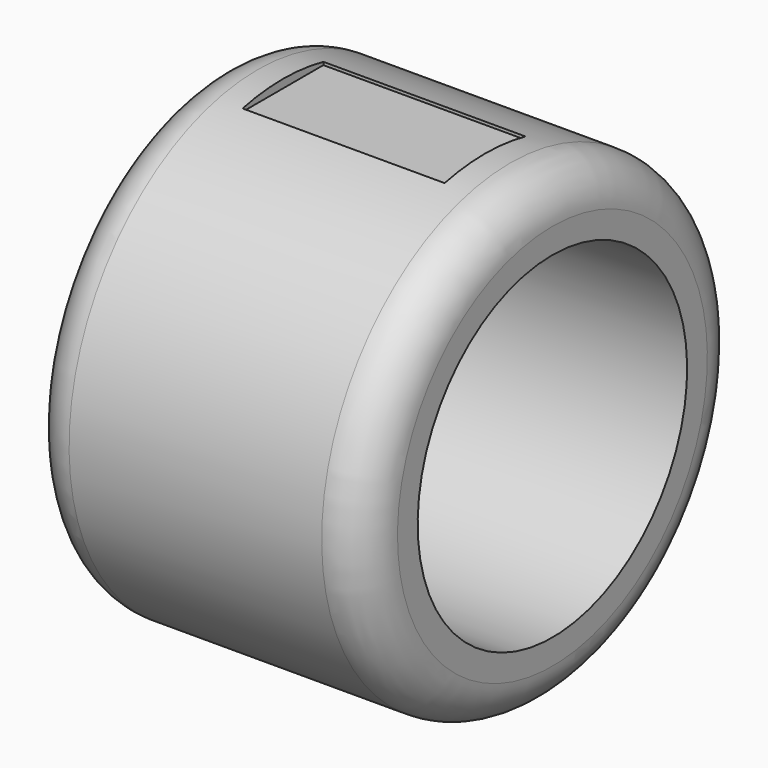
from build123d import *

# Parameters (mm, degrees)
F0_W     = 24
F0_H     = 1
F2_R     = 5
F3_DEPTH = 6


with BuildPart() as f1:
    # F0 (on Front) → F1 (revolve)
    with BuildSketch(Plane.XZ):
        Polygon((-20, 28), (-20, 20), (0, 20), (20, 20), (20, 28), (12, 28), (12, 27), (-12, 27), (-12, 28), align=None)
        with Locations((0, 27.5)):
            Rectangle(F0_W, F0_H)
    revolve(axis=Axis((2.7690531401, 0, 0), (1, 0, 0)))

    # F2
    f2_edges = [f1.edges().sort_by_distance(p)[0] for p in [
        (20, 0, -28),
        (-20, 0, -28),
    ]]
    fillet(f2_edges, radius=F2_R)

    # F0 (on Front) → F3 (cut, symmetric)
    with BuildSketch(Plane.XZ):
        with Locations((0, 27.5)):
            Rectangle(F0_W, F0_H)
    extrude(amount=F3_DEPTH, both=True, mode=Mode.SUBTRACT)


solid = f1.part
